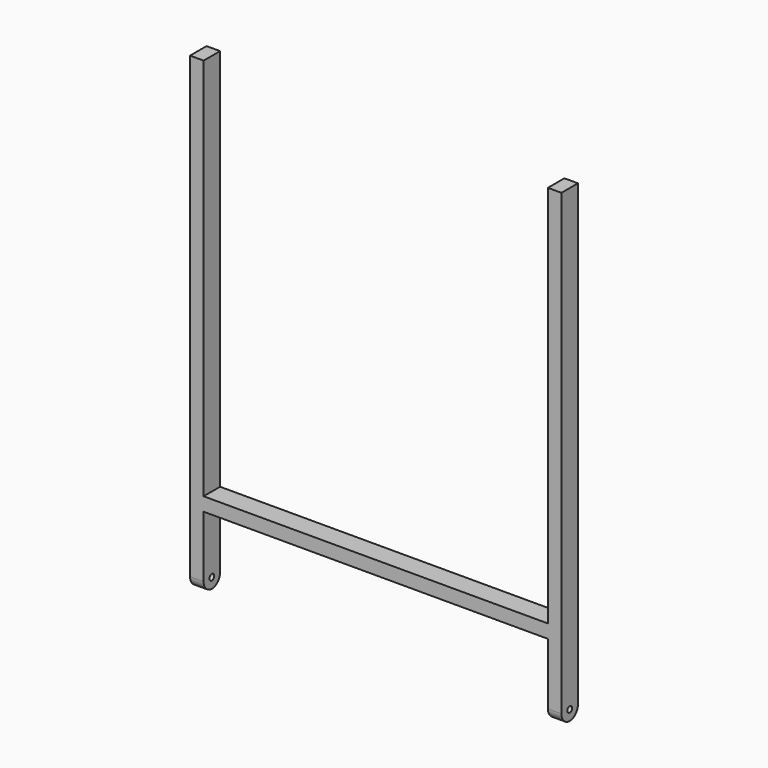
from build123d import *

# Parameters (mm, degrees)
F1_DEPTH    = 17.5
F2_R        = 2.5
F3_DEPTH    = 335
F4_T1_DEPTH = 56.5
F4_T3_DEPTH = 56.5


# Not quite as in the source:
# - a fillet or chamfer that OpenCascade refuses, or shapes differently, is made with other operations: its cross-section is extruded or revolved along the edge and cut away or added


with BuildPart() as f1:
    # F0 (on Front) → F1 (new body)
    with BuildSketch(Plane.XZ):
        Polygon((-146, -137.7746703387), (0, -137.7746703387), (146, -137.7746703387), (146, -199), (157.5, -199), (157.5, 0), (157.5, 199), (146, 199), (146, 0), (146, -126.2746703387), (8.7075978518, -126.2746703387), (0, -126.2746703387), (-6.4604924992, -126.2746703387), (-146, -126.2746703387), (-146, 0), (-146, 199), (-157.5, 199), (-157.5, 0), (-157.5, -199), (-146, -199), align=None)
    extrude(amount=F1_DEPTH)

    # F2 (on face) → F3 (cut)
    with BuildSketch(Plane(origin=(-157.5, 0, 0), x_dir=(0, -1, 0), z_dir=(-1, 0, 0))):
        with Locations((8.75, -190.25)):
            Circle(F2_R)
    extrude(amount=-F3_DEPTH, mode=Mode.SUBTRACT)

    # F4: fillet of radius 9 on 4 edges, made by hand

    # F4_s2 → F4_t1 (cut)
    with BuildSketch(Plane.YZ.offset(-180)):
        with BuildLine():
            ThreePointArc((0, -190), (-2.6360389693, -196.3639610307), (-9, -199))
            Line((-9, -199), (0, -199))
            Line((0, -199), (0, -190))
        make_face()
        with BuildLine():
            ThreePointArc((-17.5, -190), (-14.8639610307, -196.3639610307), (-8.5, -199))
            Line((-8.5, -199), (-17.5, -199))
            Line((-17.5, -199), (-17.5, -190))
        make_face()
    extrude(amount=F4_T1_DEPTH, mode=Mode.SUBTRACT)

    # F4_s4 → F4_t3 (cut)
    with BuildSketch(Plane.YZ.offset(123.5)):
        with BuildLine():
            ThreePointArc((0, -190), (-2.6360389693, -196.3639610307), (-9, -199))
            Line((-9, -199), (0, -199))
            Line((0, -199), (0, -190))
        make_face()
        with BuildLine():
            ThreePointArc((-17.5, -190), (-14.8639610307, -196.3639610307), (-8.5, -199))
            Line((-8.5, -199), (-17.5, -199))
            Line((-17.5, -199), (-17.5, -190))
        make_face()
    extrude(amount=F4_T3_DEPTH, mode=Mode.SUBTRACT)


solid = f1.part
